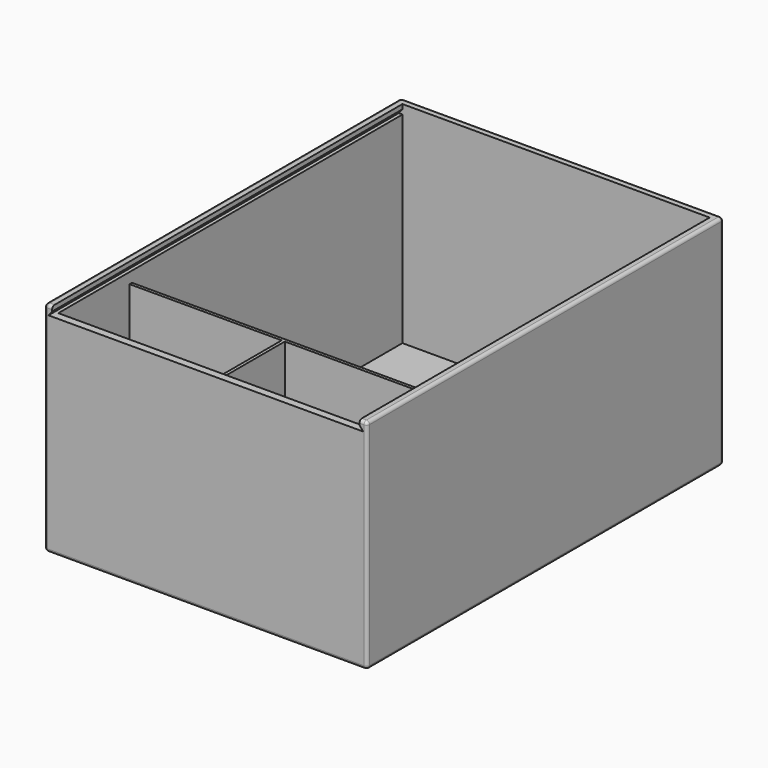
from build123d import *

# Parameters (mm, degrees)
F0_W          = 105
F0_H          = 145
F1_DEPTH      = 71
F2_T          = -2.5
F3_W          = 1
F3_H          = 29
F4_DEPTH      = 62
F5_W          = 50
F5_H          = 1.5
F6_DEPTH      = 142.5
F6_DEPTH_BACK = 268
F7_R          = 1


# Not quite as in the source:
# - an extrude ends at something that could not be found from the text; its depth is read off the source's solid


with BuildPart() as f1:
    # F0 (on Top) → F1 (new body)
    with BuildSketch(Plane.XY):
        Rectangle(F0_W, F0_H)
    extrude(amount=F1_DEPTH)

    # F2
    f2_openings = [f1.faces().sort_by_distance(p)[0] for p in [
        (0, 0, 71),
    ]]
    offset(amount=F2_T, openings=f2_openings)

    # F3 (on face) → F4 (join)
    with BuildSketch(Plane.XY.offset(2.5)):
        Polygon((-50, -40), (-50, -41), (-0.5, -41), (0.5, -41), (50, -41), (50, -40), align=None)
        with Locations((0, -55.5)):
            Rectangle(F3_W, F3_H)
    extrude(amount=F4_DEPTH)

    # F5 (on face) → F6 (cut, two sides)
    with BuildSketch(Plane.XZ.offset(72.5)) as f6_sk:
        with Locations((25, 70.25)):
            Rectangle(F5_W, F5_H)
        with Locations((-25, 70.25)):
            Rectangle(F5_W, F5_H)
        Polygon((50, 69.5), (0, 69.5), (0, 68), (51.2, 68), align=None)
        Polygon((0, 68), (0, 69.5), (-50, 69.5), (-51.2, 68), align=None)
    extrude(amount=-F6_DEPTH, mode=Mode.SUBTRACT)
    extrude(f6_sk.sketch, amount=F6_DEPTH_BACK, mode=Mode.SUBTRACT)

    # F7
    f7_edges = [f1.edges().sort_by_distance(p)[0] for p in [
        (52.5, -72.5, 35.5),
        (52.5, 72.5, 35.5),
        (52.5, 0, 0),
        (52.5, 0, 71),
        (-52.5, 72.5, 35.5),
        (-52.5, -72.5, 35.5),
        (-52.5, 0, 0),
        (-52.5, 0, 71),
        (0, 72.5, 0),
        (0, 72.5, 71),
        (0, -72.5, 0),
        (-51.25, -72.5, 71),
        (51.25, -72.5, 71),
    ]]
    fillet(f7_edges, radius=F7_R)


solid = f1.part
